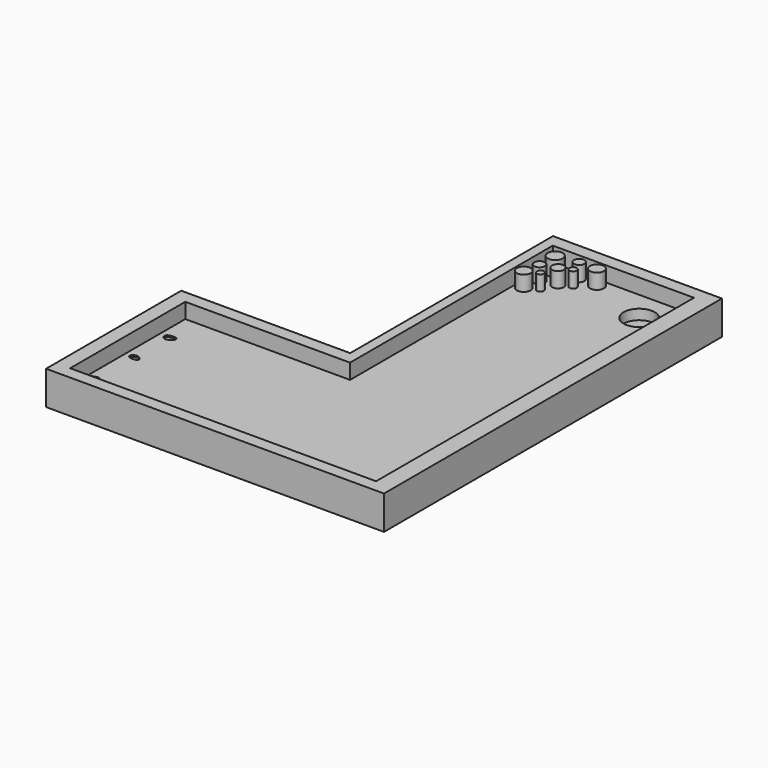
from build123d import *

# Parameters (mm, degrees)
F1_DEPTH = 10.16
F3_DEPTH = 5.08
F2_R     = 2.0763624022
F2_R_2   = 1.0345950723
F2_R_3   = 1.5897491602
F2_R_4   = 2.2416189492
F2_R_5   = 1.8002482779
F2_R_6   = 1.0905586669
F2_R_7   = 1.5614432183
F2_R_8   = 2.0977283719
F2_R_9   = 4.6843284207
F4_DEPTH = 4.572
F5_DEPTH = 7.62
F6_DEPTH = 0.762


# Not quite as in the source:
# - the program builds the solid bodies; features that only make, move or delete a surface that nothing else refers to are left out


with BuildPart() as f1:
    # F0 (on Top) → F1 (new body)
    with BuildSketch(Plane.XY):
        Polygon((47.8064281952, 65.5864290789), (-2.9935718048, 65.5864290789), (-2.9935718048, -10.6135709211), (-53.7935718048, -10.6135709211), (-53.7935718048, -61.4135709211), (47.8064281952, -61.4135709211), align=None)
    extrude(amount=F1_DEPTH)

    # F2 (on face) → F3 (cut)
    with BuildSketch(Plane.XY.offset(10.16)):
        with BuildLine():
            add(Edge.make_bspline(
                [(-47.8390082717, -23.6159972847), (-48.3000888755, -24.195855305), (-47.0430336613, -26.5169441972), (-43.1187716407, -22.9708090315), (-47.273269231, -22.904520121), (-47.8390082717, -23.6159972847)],
                knots=[0, 0, 0, 0, 0.2953373029, 0.6376255235, 1, 1, 1, 1], degree=3))
        make_face()
        with BuildLine():
            add(Edge.make_bspline(
                [(-45.2185384929, -37.5918187201), (-44.8986430919, -37.0721449164), (-46.7922945126, -35.0952494412), (-49.3003635487, -38.0785129033), (-45.5819638525, -38.1822074482), (-45.2185384929, -37.5918187201)],
                knots=[0, 0, 0, 0, 0.3255188332, 0.6301859964, 1, 1, 1, 1], degree=3))
        make_face()
        with BuildLine():
            add(Edge.make_bspline(
                [(-46.8684621155, -50.3168739378), (-46.3188154002, -50.6408562263), (-45.7691686849, -50.9648385147), (-45.2195219696, -51.2888208032)],
                knots=[0, 0, 0, 0, 1.9140753157, 1.9140753157, 1.9140753157, 1.9140753157], degree=3))
            add(Edge.make_bspline(
                [(-46.8684621155, -50.3168739378), (-47.7573276365, -50.4835154275), (-49.3321466932, -50.7787571568), (-47.6954089883, -52.20576886), (-46.1489762809, -51.633045446), (-45.2195219696, -51.2888208032)],
                knots=[0, 0, 0, 0, 0.340798916, 0.6037995791, 1, 1, 1, 1], degree=3))
        make_face()
    extrude(amount=-F3_DEPTH, mode=Mode.SUBTRACT)

    # F2 (on face) → F4 (cut)
    with BuildSketch(Plane.XY.offset(10.16)):
        with BuildLine():
            Line((0, -14.423571527), (-49.5299994946, -14.423571527))
            Line((-49.5299994946, -14.423571527), (-49.5299994946, -57.694286108))
            Line((-49.5299994946, -57.694286108), (12.2464280576, -57.694286108))
            add(Edge.make_bspline(
                [(12.2464280576, -57.694286108), (11.03689249, -55.1284041984), (8.8262402555, -50.4387756091), (16.830567108, -50.610538154), (11.543684395, -41.4140537661), (24.3541608342, -47.2929208414), (18.6630964396, -34.0142041282), (32.3027129745, -41.5037229838), (28.8060301659, -27.219324679), (39.7417437225, -32.4995208739), (41.581315462, -27.9924233376), (42.4542874098, -25.8535724133)],
                knots=[0, 0, 0, 0, 0.1112734122, 0.2033729508, 0.3034169687, 0.4180959772, 0.5306525521, 0.6520560864, 0.7731880867, 0.8923660146, 1, 1, 1, 1], degree=3))
            Line((42.4542874098, -25.8535724133), (42.4542874098, 61.7764294147))
            Line((42.4542874098, 61.7764294147), (0, 61.7764294147))
            Line((0, 61.7764294147), (0, -14.423571527))
        make_face()
        with BuildLine():
            add(Edge.make_bspline(
                [(-46.8684621155, -50.3168739378), (-47.7573276365, -50.4835154275), (-49.3321466932, -50.7787571568), (-47.6954089883, -52.20576886), (-46.1489762809, -51.633045446), (-45.2195219696, -51.2888208032)],
                knots=[0, 0, 0, 0, 0.340798916, 0.6037995791, 1, 1, 1, 1], degree=3))
            add(Edge.make_bspline(
                [(-46.8684621155, -50.3168739378), (-46.3188154002, -50.6408562263), (-45.7691686849, -50.9648385147), (-45.2195219696, -51.2888208032)],
                knots=[0, 0, 0, 0, 1.9140753157, 1.9140753157, 1.9140753157, 1.9140753157], degree=3))
        make_face(mode=Mode.SUBTRACT)
        with BuildLine():
            add(Edge.make_bspline(
                [(-45.2185384929, -37.5918187201), (-44.8986430919, -37.0721449164), (-46.7922945126, -35.0952494412), (-49.3003635487, -38.0785129033), (-45.5819638525, -38.1822074482), (-45.2185384929, -37.5918187201)],
                knots=[0, 0, 0, 0, 0.3255188332, 0.6301859964, 1, 1, 1, 1], degree=3))
        make_face(mode=Mode.SUBTRACT)
        with BuildLine():
            add(Edge.make_bspline(
                [(-47.8390082717, -23.6159972847), (-48.3000888755, -24.195855305), (-47.0430336613, -26.5169441972), (-43.1187716407, -22.9708090315), (-47.273269231, -22.904520121), (-47.8390082717, -23.6159972847)],
                knots=[0, 0, 0, 0, 0.2953373029, 0.6376255235, 1, 1, 1, 1], degree=3))
        make_face(mode=Mode.SUBTRACT)
        with Locations((2.6250390802, 47.6025752723)):
            Circle(F2_R, mode=Mode.SUBTRACT)
        with Locations((6.2461188063, 49.3268966675)):
            Circle(F2_R_2, mode=Mode.SUBTRACT)
        with Locations((3.4872009419, 52.4306818843)):
            Circle(F2_R_3, mode=Mode.SUBTRACT)
        with Locations((3.6596332211, 58.1209473312)):
            Circle(F2_R_4, mode=Mode.SUBTRACT)
        with Locations((7.9704420641, 53.8101382554)):
            Circle(F2_R_5, mode=Mode.SUBTRACT)
        with Locations((11.2466607243, 55.3620308638)):
            Circle(F2_R_6, mode=Mode.SUBTRACT)
        with Locations((10.0396340713, 59.1555424035)):
            Circle(F2_R_7, mode=Mode.SUBTRACT)
        with Locations((15.3850372881, 59.1555424035)):
            Circle(F2_R_8, mode=Mode.SUBTRACT)
        with Locations((33.3180055022, 52.6031143963)):
            Circle(F2_R_9, mode=Mode.SUBTRACT)
        with BuildLine():
            add(Edge.make_bspline(
                [(12.2464280576, -57.694286108), (11.03689249, -55.1284041984), (8.8262402555, -50.4387756091), (16.830567108, -50.610538154), (11.543684395, -41.4140537661), (24.3541608342, -47.2929208414), (18.6630964396, -34.0142041282), (32.3027129745, -41.5037229838), (28.8060301659, -27.219324679), (39.7417437225, -32.4995208739), (41.581315462, -27.9924233376), (42.4542874098, -25.8535724133)],
                knots=[0, 0, 0, 0, 0.1112734122, 0.2033729508, 0.3034169687, 0.4180959772, 0.5306525521, 0.6520560864, 0.7731880867, 0.8923660146, 1, 1, 1, 1], degree=3))
            Line((12.2464280576, -57.694286108), (42.4542874098, -57.694286108))
            Line((42.4542874098, -57.694286108), (42.4542874098, -25.8535724133))
        make_face()
    extrude(amount=-F4_DEPTH, mode=Mode.SUBTRACT)

    # F5 (cut): a face of the model
    f5_faces = [f1.faces().sort_by_distance(p)[0] for p in [
        (33.3180055022, 52.6031143963, 10.16),
    ]]
    extrude(f5_faces, amount=-F5_DEPTH, mode=Mode.SUBTRACT)

    # F2 (on face) → F6 (cut)
    with BuildSketch(Plane.XY.offset(10.16)):
        with BuildLine():
            add(Edge.make_bspline(
                [(12.2464280576, -57.694286108), (11.03689249, -55.1284041984), (8.8262402555, -50.4387756091), (16.830567108, -50.610538154), (11.543684395, -41.4140537661), (24.3541608342, -47.2929208414), (18.6630964396, -34.0142041282), (32.3027129745, -41.5037229838), (28.8060301659, -27.219324679), (39.7417437225, -32.4995208739), (41.581315462, -27.9924233376), (42.4542874098, -25.8535724133)],
                knots=[0, 0, 0, 0, 0.1112734122, 0.2033729508, 0.3034169687, 0.4180959772, 0.5306525521, 0.6520560864, 0.7731880867, 0.8923660146, 1, 1, 1, 1], degree=3))
            Line((12.2464280576, -57.694286108), (42.4542874098, -57.694286108))
            Line((42.4542874098, -57.694286108), (42.4542874098, -25.8535724133))
        make_face()
    extrude(amount=-F6_DEPTH, mode=Mode.SUBTRACT)


solid = f1.part
